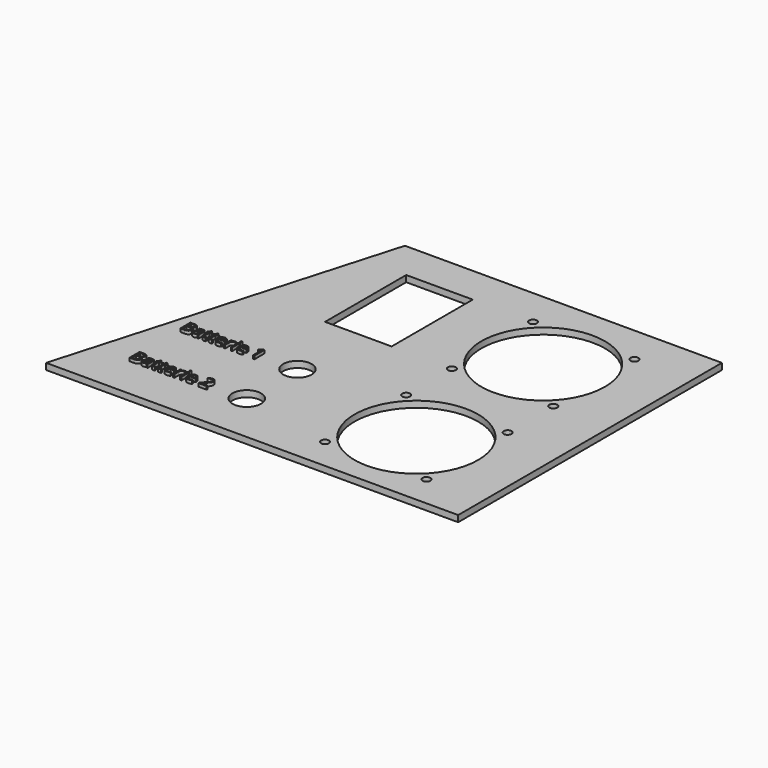
from build123d import *

# Parameters (mm, degrees)
F0_R         = 4.5
F0_R_2       = 19.5
F0_W         = 21
F0_H         = 32
F1_DEPTH     = 2
F2_D         = 2.5
F3_TEXT_SIZE = 5.5555555556
F4_DEPTH     = 3


# Not quite as in the source:
# - Text() gives the source's letters only with a copy of the font that has no kerning and outlines rounded to 1/6400 em; it was checked with that copy


with BuildPart() as f1:
    # F0 (on Top) → F1 (new body)
    with BuildSketch(Plane.XY):
        Polygon((30, 104), (0, 0), (130, 0), (130, 104), align=None)
        with Locations((50.5, 16)):
            Circle(F0_R, mode=Mode.SUBTRACT)
        with Locations((50.5, 36)):
            Circle(F0_R, mode=Mode.SUBTRACT)
        with Locations((96, 26)):
            Circle(F0_R_2, mode=Mode.SUBTRACT)
        with Locations((50.5, 76)):
            Rectangle(F0_W, F0_H, mode=Mode.SUBTRACT)
        with Locations((96, 76)):
            Circle(F0_R_2, mode=Mode.SUBTRACT)
    extrude(amount=F1_DEPTH)

    # F2 (through all)
    with Locations(Plane(origin=(0, 0, 0), x_dir=(1, 0, 0), z_dir=(0, 0, -1))):
        with Locations((112, -92), (80, -92), (80, -60), (112, -60), (112, -42), (80, -42), (80, -10), (112, -10)):
            Hole(F2_D / 2)

    # F3 (on Top) → F4 (join)
    with BuildSketch(Plane.XY):
        with Locations((15, 33.5)):
            Text('Batterie 1', F3_TEXT_SIZE, font='Open Sans', text_align=(TextAlign.LEFT, TextAlign.BOTTOM))
        with Locations((15, 13.5)):
            Text('Batterie 2', F3_TEXT_SIZE, font='Open Sans', text_align=(TextAlign.LEFT, TextAlign.BOTTOM))
    extrude(amount=F4_DEPTH)


solid = f1.part
